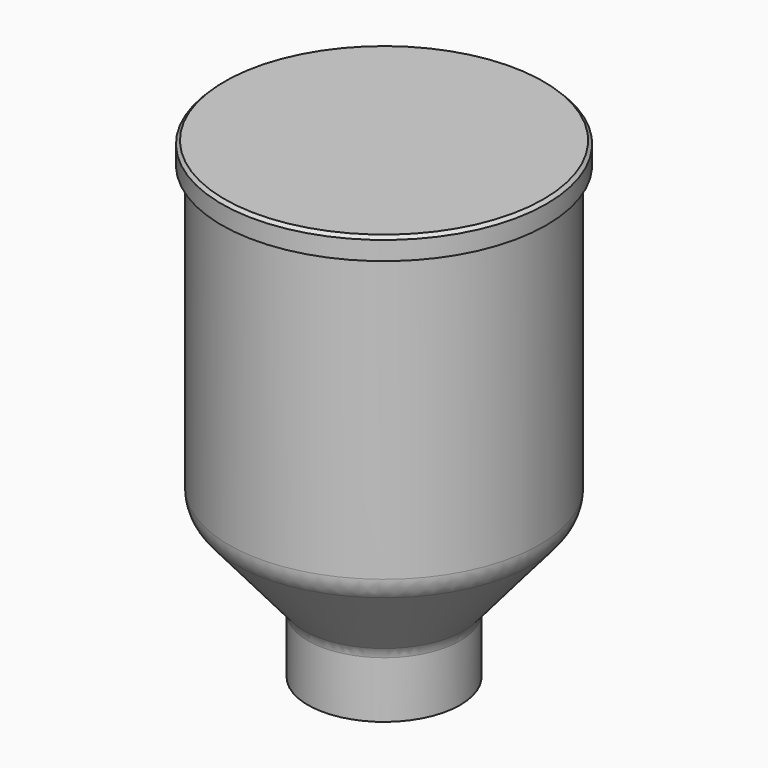
from build123d import *

# Parameters (mm, degrees)
F0_R      = 24.5
F1_DEPTH  = 20
F1_FACE_R = 24.5
F3_R      = 50
F5_DEPTH  = 100
F6_R      = 5
F7_R      = 10
F8_T      = -1
F9_R      = 52.3
F9_R_2    = 50.3
F9_R_3    = 50
F9_R_4    = 49
F10_DEPTH = 2
F11_DEPTH = 5
F12_SIZE  = 1
F13_SIZE  = 0.6


with BuildPart() as f1:
    # F0 (on Top) → F1 (new body)
    with BuildSketch(Plane.XY):
        Circle(F0_R)
    extrude(amount=F1_DEPTH)

    # F1_face (on face) → F4 section 0
    with BuildSketch(Plane.XY.offset(20)):
        Circle(F1_FACE_R)
    # F3 (on offset) → F4 section 1
    with BuildSketch(Plane.XY.offset(50)):
        Circle(F3_R)
    loft()

    # F5 (add): a face of the model
    f5_faces = [f1.faces().sort_by_distance(p)[0] for p in [
        (0, 0, 50),
    ]]
    extrude(f5_faces, amount=F5_DEPTH)

    # F6
    f6_edges = [f1.edges().sort_by_distance(p)[0] for p in [
        (-24.5, 0, 20),
    ]]
    fillet(f6_edges, radius=F6_R)

    # F7
    f7_edges = [f1.edges().sort_by_distance(p)[0] for p in [
        (-50, 0, 50),
    ]]
    fillet(f7_edges, radius=F7_R)

    # F8
    f8_openings = [f1.faces().sort_by_distance(p)[0] for p in [
        (0, 0, 0),
        (0, 0, 150),
    ]]
    offset(amount=F8_T, openings=f8_openings)


with BuildPart() as f10:
    # F9 (on face) → F10 (new body)
    with BuildSketch(Plane.XY.offset(150)):
        Circle(F9_R)
        Circle(F9_R_2, mode=Mode.SUBTRACT)
        Circle(F9_R_2)
        Circle(F9_R_3, mode=Mode.SUBTRACT)
        Circle(F9_R_3)
        Circle(F9_R_4, mode=Mode.SUBTRACT)
        Circle(F9_R_4)
    extrude(amount=F10_DEPTH)

    # F9 (on face) → F11 (join)
    with BuildSketch(Plane.XY.offset(150)):
        Circle(F9_R)
        Circle(F9_R_2, mode=Mode.SUBTRACT)
    extrude(amount=-F11_DEPTH)

    # F12
    f12_edges = [f10.edges().sort_by_distance(p)[0] for p in [
        (-52.3, 0, 152),
    ]]
    chamfer(f12_edges, length=F12_SIZE)

    # F13
    f13_edges = [f10.edges().sort_by_distance(p)[0] for p in [
        (-50.3, 0, 145),
    ]]
    chamfer(f13_edges, length=F13_SIZE)


solid = Compound([f1.part, f10.part])
